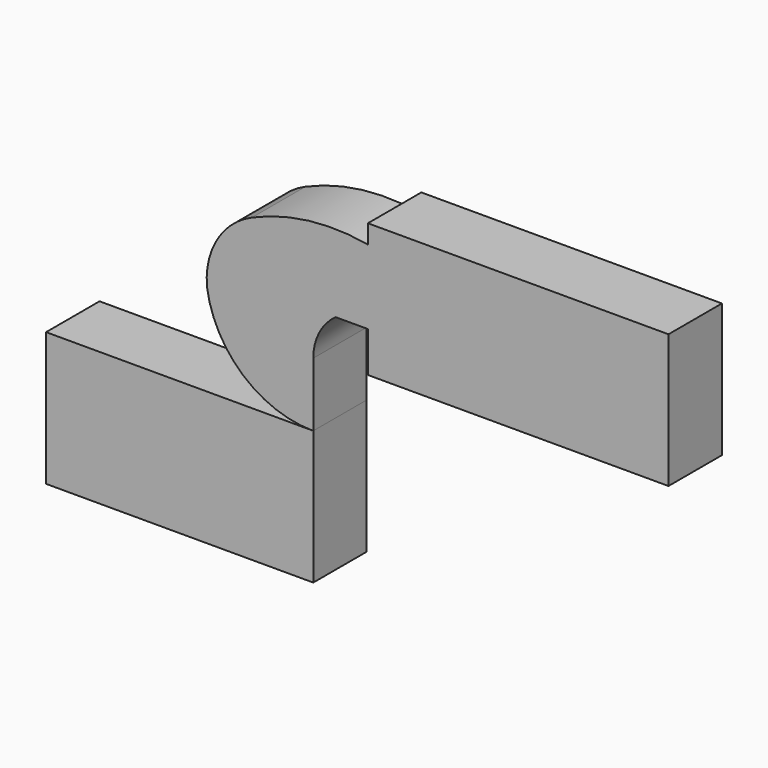
from build123d import *

# Parameters (mm, degrees)
F1_DEPTH = 25.4
F0_W     = 101.6
F0_H     = 50.8


with BuildPart() as f1:
    # F0 (on Front) → F1 (new body)
    with BuildSketch(Plane.XZ):
        with BuildLine():
            ThreePointArc((10.3944045648, 60.3657866119), (24.082878262, 35.3551021018), (50.8, 25.4))
            Line((50.8, 25.4), (50.8, 38.0313412011))
            Line((50.8, 38.0313412011), (50.8, 49.7220940888))
            ThreePointArc((50.8, 49.7220940888), (53.0487528423, 59.0045752006), (59.2963695526, 66.2287450752))
            Line((59.2963695526, 66.2287450752), (71.5682441892, 66.2287450752))
            Line((71.5682441892, 66.2287450752), (71.5682441892, 94.4982363395))
            ThreePointArc((71.5682441892, 94.4982363395), (49.1341654269, 95.1751720147), (27.4917148054, 89.2295464873))
            ThreePointArc((27.4917148054, 89.2295464873), (14.2628571936, 77.5699621317), (10.3944045648, 60.3657866119))
        make_face()
        with BuildLine():
            ThreePointArc((117.9655272715, 66.2287450752), (97.3968675917, 84.6799466274), (71.5682441892, 94.4982363395))
            Line((71.5682441892, 94.4982363395), (71.5682441892, 66.2287450752))
            Line((71.5682441892, 66.2287450752), (117.9655272715, 66.2287450752))
        make_face()
        with BuildLine():
            Line((71.5682441892, 101.6453287184), (71.5682441892, 94.4982363395))
            ThreePointArc((71.5682441892, 94.4982363395), (97.3968675917, 84.6799466274), (117.9655272715, 66.2287450752))
            Line((117.9655272715, 66.2287450752), (71.5682441892, 66.2287450752))
            Line((71.5682441892, 66.2287450752), (71.5682441892, 50.8453287184))
            Line((71.5682441892, 50.8453287184), (185.8682441892, 50.8453287184))
            Line((185.8682441892, 50.8453287184), (185.8682441892, 101.6453287184))
            Line((185.8682441892, 101.6453287184), (71.5682441892, 101.6453287184))
        make_face()
    extrude(amount=F1_DEPTH)


with BuildPart() as f1b:
    # F0 (on Front) → F1, piece 2 (new body)
    with BuildSketch(Plane.XZ):
        Rectangle(F0_W, F0_H)
    extrude(amount=F1_DEPTH)


solid = Compound([f1.part, f1b.part])
